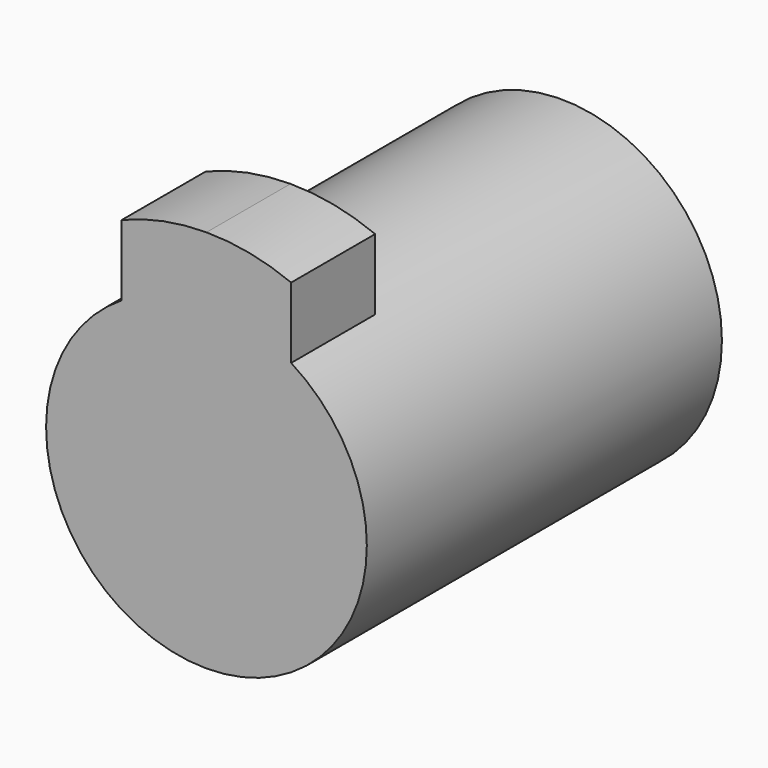
from build123d import *

# Parameters (mm, degrees)
F0_R     = 18.034
F1_DEPTH = 49.911
F3_DEPTH = 11.811
F5_DEPTH = 14.224


with BuildPart() as f1:
    # F0 (on Front) → F1 (new body)
    with BuildSketch(Plane.XZ):
        Circle(F0_R)
    extrude(amount=-F1_DEPTH)

    # F2 (on Front) → F3 (join)
    with BuildSketch(Plane.XZ):
        with BuildLine():
            ThreePointArc((-9.525, 15.3133775177), (0, 18.034), (9.525, 15.3133775177))
            Line((9.525, 15.3133775177), (9.525, 23.2722085544))
            ThreePointArc((9.525, 23.2722085544), (4.8537799544, 24.6731055231), (0, 25.146))
            ThreePointArc((0, 25.146), (-4.8537799544, 24.6731055231), (-9.525, 23.2722085544))
            Line((-9.525, 23.2722085544), (-9.525, 15.3133775177))
        make_face()
    extrude(amount=-F3_DEPTH)

    # F4 (on face) → F5 (join)
    with BuildSketch(Plane(origin=(0, 49.911, 0), x_dir=(-1, 0, 0), z_dir=(0, 1, 0))):
        with BuildLine():
            Line((1.0317528774, 1.2065), (-1.0317528774, 1.2065))
            ThreePointArc((-1.0317528774, 1.2065), (0, -1.5875), (1.0317528774, 1.2065))
        make_face()
    extrude(amount=F5_DEPTH)


solid = f1.part
